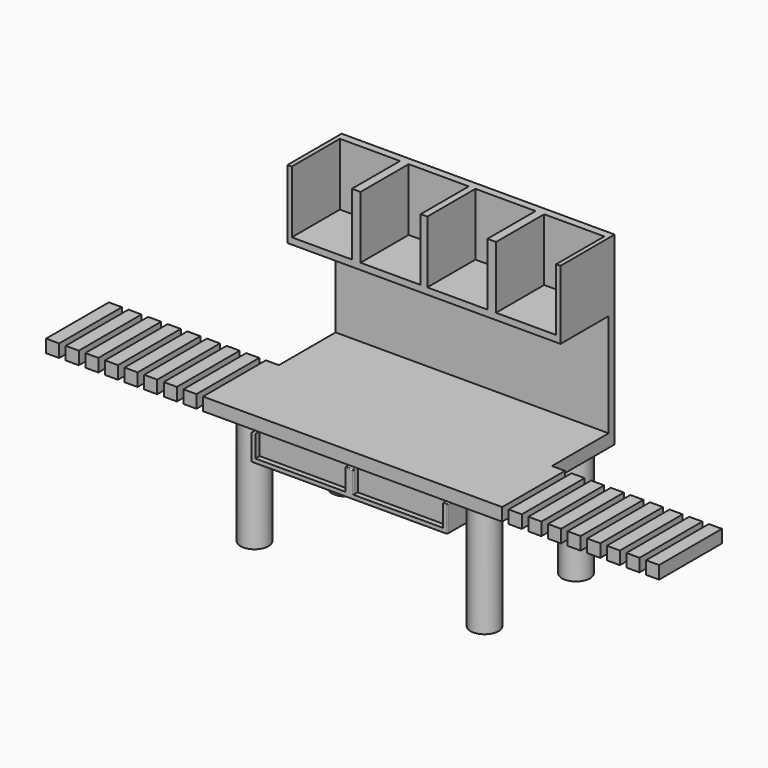
from build123d import *

# Parameters (mm, degrees)
F0_W           = 77.3143488
F0_H           = 463.8860572777
F0_W_2         = 77.3143428796
F1_DEPTH       = 76.2
F2_W           = 1613.9369076119
F2_H           = 400.3860572777
F3_DEPTH       = 1016
F4_R           = 82.55
F5_DEPTH       = 660.4
F6_W           = 1613.9369076119
F6_H           = 609.6
F7_DEPTH       = 355.6
F8_W           = 355.6
F8_H           = 368.3
F9_DEPTH       = 355.6
F10_W          = 1158.9655992915
F10_H          = 152.4
F11_DEPTH      = 304.8
F11_DEPTH_BACK = 25.4
F12_W          = 528.6827996458
F12_H          = 128.8552815199
F13_DEPTH      = 31.75
F14_R          = 5.08


# Not quite as in the source:
# - two fillets or chamfers of one size are made in one step


with BuildPart() as f1:
    # F0 (on Top) → F1 (new body)
    with BuildSketch(Plane.XY):
        Polygon((0, 463.8860572777), (0, 0), (1613.9369076119, 0), (1613.9369076119, 463.8860572777), (1613.9369076119, 927.7721145553), (0, 927.7721145553), align=None)
        with Locations((-38.6571744, 231.9430286388)):
            Rectangle(F0_W, F0_H)
        with Locations((1652.5940790517, 231.9430286388)):
            Rectangle(F0_W_2, F0_H)
    extrude(amount=-F1_DEPTH)

    # F2 (on face) → F3 (join)
    with BuildSketch(Plane.XY):
        with Locations((806.968453806, 727.5790859165)):
            Rectangle(F2_W, F2_H)
    extrude(amount=F3_DEPTH)

    # F4 (on face) → F5 (join)
    with BuildSketch(Plane(origin=(0, 0, -76.2), x_dir=(1, 0, 0), z_dir=(0, 0, -1))):
        with Locations((127, -800.7721145553)):
            Circle(F4_R)
        with Locations((1486.9369076119, -800.7721145553)):
            Circle(F4_R)
        with Locations((127, -125.1321285963)):
            Circle(F4_R)
        with Locations((1486.9369016915, -125.1321285963)):
            Circle(F4_R)
    extrude(amount=F5_DEPTH)

    # F6 (on face) → F7 (cut)
    with BuildSketch(Plane.XZ.offset(-527.3860572777)):
        with Locations((806.968453806, 304.8)):
            Rectangle(F6_W, F6_H)
    extrude(amount=-F7_DEPTH, mode=Mode.SUBTRACT)

    # F8 (on face) → F9 (cut)
    with BuildSketch(Plane.XZ.offset(-527.3860572777)):
        with Locations((203.2, 831.85)):
            Rectangle(F8_W, F8_H)
        with Locations((609.6, 831.85)):
            Rectangle(F8_W, F8_H)
        with Locations((1004.3369076119, 831.85)):
            Rectangle(F8_W, F8_H)
        with Locations((1410.7369076119, 831.85)):
            Rectangle(F8_W, F8_H)
    extrude(amount=-F9_DEPTH, mode=Mode.SUBTRACT)

    # F10 (on face) → F11 (join, two sides)
    with BuildSketch(Plane.XZ) as f11_sk:
        with Locations((806.9684508458, -152.4)):
            Rectangle(F10_W, F10_H)
    extrude(amount=-F11_DEPTH)
    extrude(f11_sk.sketch, amount=F11_DEPTH_BACK)

    # F12 (on face) → F13 (cut)
    with BuildSketch(Plane.XZ.offset(25.4)):
        with Locations((517.2270510229, -140.6276407599)):
            Rectangle(F12_W, F12_H)
        with Locations((1096.7098506686, -140.6276407599)):
            Rectangle(F12_W, F12_H)
    extrude(amount=-F13_DEPTH, mode=Mode.SUBTRACT)

    # F14
    f14_edges = [f1.edges().sort_by_distance(p)[0] for p in [
        (240.185651, -25.4, -76.2),
        (227.485651, -25.4, -152.4),
        (1386.45125, -12.7, -76.2),
        (1386.45125, -25.4, -152.4),
        (227.485651, -12.7, -76.2),
        (832.368451, -12.7, -76.2),
        (806.968451, -25.4, -76.2),
        (781.568451, -12.7, -76.2),
        (1373.75125, -25.4, -76.2),
        (781.568451, -25.4, -140.627641),
        (832.368451, -25.4, -140.627641),
    ]]
    fillet(f14_edges, radius=F14_R)


with BuildPart() as f1b:
    # F0 (on Top) → F1, piece 2 (new body)
    with BuildSketch(Plane.XY):
        with Locations((1768.5655933711, 231.9430286388)):
            Rectangle(F0_W_2, F0_H)
    extrude(amount=-F1_DEPTH)


with BuildPart() as f1c:
    # F0 (on Top) → F1, piece 3 (new body)
    with BuildSketch(Plane.XY):
        with Locations((1884.5371076906, 231.9430286388)):
            Rectangle(F0_W_2, F0_H)
    extrude(amount=-F1_DEPTH)


with BuildPart() as f1d:
    # F0 (on Top) → F1, piece 4 (new body)
    with BuildSketch(Plane.XY):
        with Locations((2000.50862201, 231.9430286388)):
            Rectangle(F0_W_2, F0_H)
    extrude(amount=-F1_DEPTH)


with BuildPart() as f1e:
    # F0 (on Top) → F1, piece 5 (new body)
    with BuildSketch(Plane.XY):
        with Locations((2116.4801363294, 231.9430286388)):
            Rectangle(F0_W_2, F0_H)
    extrude(amount=-F1_DEPTH)


with BuildPart() as f1f:
    # F0 (on Top) → F1, piece 6 (new body)
    with BuildSketch(Plane.XY):
        with Locations((2232.4516506488, 231.9430286388)):
            Rectangle(F0_W_2, F0_H)
    extrude(amount=-F1_DEPTH)


with BuildPart() as f1g:
    # F0 (on Top) → F1, piece 7 (new body)
    with BuildSketch(Plane.XY):
        with Locations((2348.4231649682, 231.9430286388)):
            Rectangle(F0_W_2, F0_H)
    extrude(amount=-F1_DEPTH)


with BuildPart() as f1h:
    # F0 (on Top) → F1, piece 8 (new body)
    with BuildSketch(Plane.XY):
        with Locations((2464.3946792876, 231.9430286388)):
            Rectangle(F0_W_2, F0_H)
    extrude(amount=-F1_DEPTH)


with BuildPart() as f1i:
    # F0 (on Top) → F1, piece 9 (new body)
    with BuildSketch(Plane.XY):
        with Locations((2580.3661936071, 231.9430286388)):
            Rectangle(F0_W_2, F0_H)
    extrude(amount=-F1_DEPTH)


with BuildPart() as f1j:
    # F0 (on Top) → F1, piece 10 (new body)
    with BuildSketch(Plane.XY):
        with Locations((-966.4292948757, 231.9430286388)):
            Rectangle(F0_W_2, F0_H)
    extrude(amount=-F1_DEPTH)


with BuildPart() as f1k:
    # F0 (on Top) → F1, piece 11 (new body)
    with BuildSketch(Plane.XY):
        with Locations((-850.4577805563, 231.9430286388)):
            Rectangle(F0_W_2, F0_H)
    extrude(amount=-F1_DEPTH)


with BuildPart() as f1l:
    # F0 (on Top) → F1, piece 12 (new body)
    with BuildSketch(Plane.XY):
        with Locations((-734.4862662369, 231.9430286388)):
            Rectangle(F0_W_2, F0_H)
    extrude(amount=-F1_DEPTH)


with BuildPart() as f1m:
    # F0 (on Top) → F1, piece 13 (new body)
    with BuildSketch(Plane.XY):
        with Locations((-618.5147519175, 231.9430286388)):
            Rectangle(F0_W_2, F0_H)
    extrude(amount=-F1_DEPTH)


with BuildPart() as f1n:
    # F0 (on Top) → F1, piece 14 (new body)
    with BuildSketch(Plane.XY):
        with Locations((-502.5432375981, 231.9430286388)):
            Rectangle(F0_W_2, F0_H)
    extrude(amount=-F1_DEPTH)


with BuildPart() as f1o:
    # F0 (on Top) → F1, piece 15 (new body)
    with BuildSketch(Plane.XY):
        with Locations((-386.5717232786, 231.9430286388)):
            Rectangle(F0_W_2, F0_H)
    extrude(amount=-F1_DEPTH)


with BuildPart() as f1p:
    # F0 (on Top) → F1, piece 16 (new body)
    with BuildSketch(Plane.XY):
        with Locations((-270.6002089592, 231.9430286388)):
            Rectangle(F0_W_2, F0_H)
    extrude(amount=-F1_DEPTH)


with BuildPart() as f1q:
    # F0 (on Top) → F1, piece 17 (new body)
    with BuildSketch(Plane.XY):
        with Locations((-154.6286946398, 231.9430286388)):
            Rectangle(F0_W_2, F0_H)
    extrude(amount=-F1_DEPTH)


solid = Compound([f1.part, f1b.part, f1c.part, f1d.part, f1e.part, f1f.part, f1g.part, f1h.part, f1i.part, f1j.part, f1k.part, f1l.part, f1m.part, f1n.part, f1o.part, f1p.part, f1q.part])
